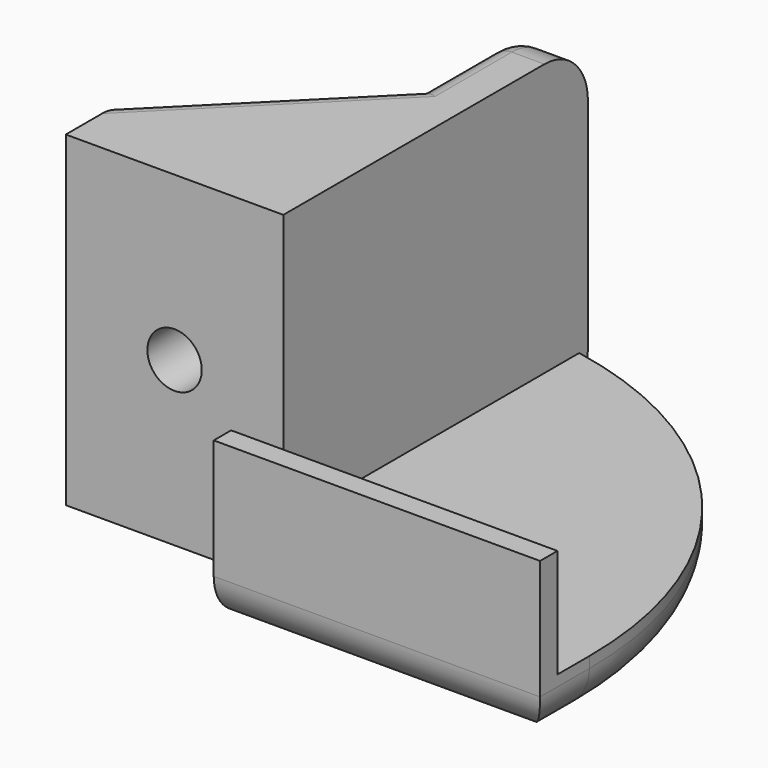
from build123d import *

# Parameters (mm, degrees)
F0_W          = 30
F0_H          = 42
F1_DEPTH      = 5
F2_T1_DEPTH   = 186.6590212458
F3_W          = 30
F3_H          = 2
F4_DEPTH      = 10
F5_W          = 35
F5_H          = 30
F6_DEPTH      = 5
F7_W          = 7
F7_H          = 30
F8_DEPTH      = 15
F9_R          = 2.5
F10_DEPTH     = 10
F11_R         = 4
F12_W         = 15
F12_H         = 14
F13_DEPTH     = 5
F14_W         = 15
F14_H         = 15
F15_DEPTH     = 5
F16_T4_DEPTH  = 35.8601958556
F16_T9_DEPTH  = 35.8601958556
F17_R         = 5
F18_T1_DEPTH  = 20
F18_T6_DEPTH  = 9.5699020722
F18_T11_DEPTH = 31.2132034356
F18_T16_DEPTH = 31.2132034356
F18_T21_DEPTH = 14
F18_T24_ANGLE = 90
F18_T26_ANGLE = 90
F18_T30_DEPTH = 13
F18_T36_DEPTH = 14
F18_T40_DEPTH = 31.2132034356
F18_T47_DEPTH = 13
F18_T51_DEPTH = 31.2132034356


# Not quite as in the source:
# - a fillet or chamfer that OpenCascade refuses, or shapes differently, is made with other operations: its cross-section is extruded or revolved along the edge and cut away or added


with BuildPart() as f1:
    # F0 (on Top) → F1 (new body)
    with BuildSketch(Plane.XY):
        with Locations((15, 21)):
            Rectangle(F0_W, F0_H)
    extrude(amount=F1_DEPTH)

    # F2: fillet of radius 37 on 1 edges, made by hand

    # F2_s2 → F2_t1 (cut)
    with BuildSketch(Plane.XY.offset(-90.8295106229)):
        with BuildLine():
            ThreePointArc((30, 5.6681957508), (21.5306852354, 29.2266337296), (0, 42))
            Line((0, 42), (30, 42))
            Line((30, 42), (30, 5.6681957508))
        make_face()
    extrude(amount=F2_T1_DEPTH, mode=Mode.SUBTRACT)

    # F3 (on face) → F4 (join)
    with BuildSketch(Plane.XY.offset(5)):
        with Locations((15, 1)):
            Rectangle(F3_W, F3_H)
    extrude(amount=F4_DEPTH)

    # F5 (on face) → F6 (join)
    with BuildSketch(Plane(origin=(0, 0, 0), x_dir=(0, -1, 0), z_dir=(-1, 0, 0))):
        with Locations((-25.5, 15)):
            Rectangle(F5_W, F5_H)
    extrude(amount=F6_DEPTH)

    # F7 (on face) → F8 (join)
    with BuildSketch(Plane(origin=(-5, 0, 0), x_dir=(0, -1, 0), z_dir=(-1, 0, 0))):
        with Locations((-11.5, 15)):
            Rectangle(F7_W, F7_H)
    extrude(amount=F8_DEPTH)

    # F9 (on face) → F10 (cut)
    with BuildSketch(Plane(origin=(0, 15, 0), x_dir=(-1, 0, 0), z_dir=(0, 1, 0))):
        with Locations((10, 15)):
            Circle(F9_R)
    extrude(amount=-F10_DEPTH, mode=Mode.SUBTRACT)

    # F11
    f11_edges = [f1.edges().sort_by_distance(p)[0] for p in [
        (21.530685, 29.226634, 0),
        (15, 0, 0),
    ]]
    fillet(f11_edges, radius=F11_R)

    # F12 (on face) → F13 (join)
    with BuildSketch(Plane(origin=(0, 0, 0), x_dir=(1, 0, 0), z_dir=(0, 0, -1))):
        with Locations((-12.5, -22)):
            Rectangle(F12_W, F12_H)
    extrude(amount=-F13_DEPTH)

    # F14 (on face) → F15 (join)
    with BuildSketch(Plane.XY.offset(30)):
        with Locations((-12.5, 22.5)):
            Rectangle(F14_W, F14_H)
    extrude(amount=-F15_DEPTH)

    # F16: chamfer of 15 on 2 edges, made by hand


with BuildPart() as f16_tool2:
    # F16_s3 → F16_t4 (new body)
    with BuildSketch(Plane.XY.offset(45.4300979278)):
        with BuildLine():
            Line((-20.4242640687, 14.5757359313), (-4.5757359313, 30.4242640687))
            Line((-4.5757359313, 30.4242640687), (-4.5757359313, 30.7242640687))
            ThreePointArc((-4.5757359313, 30.7242640687), (-12.2878679656, 30.3), (-20, 30.3))
            Line((-20, 30.3), (-20.3, 30))
            ThreePointArc((-20.3, 30), (-20.3, 22.2878679656), (-20.7242640687, 14.5757359313))
            Line((-20.7242640687, 14.5757359313), (-20.4242640687, 14.5757359313))
        make_face()
    extrude(amount=-F16_T4_DEPTH)

    split(bisect_by=Plane.YZ.offset(-5), keep=Keep.BOTTOM)


with BuildPart() as f1_1:
    add(f1.part)

    # F16_t1: cut F16_tool2
    add(f16_tool2.part, mode=Mode.SUBTRACT)


with BuildPart() as f16_tool7:
    # F16_s8 → F16_t9 (new body)
    with BuildSketch(Plane.XY.offset(-15.4300979278)):
        with BuildLine():
            Line((-4.5757359313, 29.4242640687), (-20.4242640687, 13.5757359313))
            Line((-20.4242640687, 13.5757359313), (-20.7242640687, 13.5757359313))
            ThreePointArc((-20.7242640687, 13.5757359313), (-20.3, 21.2878679656), (-20.3, 29))
            Line((-20.3, 29), (-20, 29.3))
            ThreePointArc((-20, 29.3), (-12.2878679656, 29.3), (-4.5757359313, 29.7242640687))
            Line((-4.5757359313, 29.7242640687), (-4.5757359313, 29.4242640687))
        make_face()
    extrude(amount=F16_T9_DEPTH)

    split(bisect_by=Plane.YZ.offset(-5), keep=Keep.BOTTOM)


with BuildPart() as f1_2:
    add(f1_1.part)

    # F16_t6: cut F16_tool7
    add(f16_tool7.part, mode=Mode.SUBTRACT)

    # F17
    f17_edges = [f1_2.edges().sort_by_distance(p)[0] for p in [
        (-2.5, 43, 0),
        (-2.5, 43, 30),
    ]]
    fillet(f17_edges, radius=F17_R)

    # F18: fillet of radius 2 on 9 edges, made by hand

    # F18_s2 → F18_t1 (cut)
    with BuildSketch(Plane.XY.offset(5)):
        with BuildLine():
            ThreePointArc((-3, 43), (-4.4142135624, 42.4142135624), (-5, 41))
            Line((-5, 41), (-5, 43))
            Line((-5, 43), (-3, 43))
        make_face()
    extrude(amount=F18_T1_DEPTH, mode=Mode.SUBTRACT)


with BuildPart() as f18_tool4:
    # F18_s5 → F18_t6 (new body)
    with BuildSketch(Plane.XY.offset(25)):
        with BuildLine():
            ThreePointArc((-20, 13), (-19.4142135624, 14.4142135624), (-18, 15))
            Line((-18, 15), (-20, 15))
            Line((-20, 15), (-20, 13))
        make_face()
    extrude(amount=-F18_T6_DEPTH)

    split(bisect_by=Plane(origin=(-17, 17, 0), x_dir=(0, 0, 1), z_dir=(-0.7071067812, 0.7071067812, 0)), keep=Keep.TOP)


with BuildPart() as f1_3:
    add(f1_2.part)

    # F18_t3: cut F18_tool4
    add(f18_tool4.part, mode=Mode.SUBTRACT)


with BuildPart() as f18_tool9:
    # F18_s10 → F18_t11 (new body)
    with BuildSketch(Plane(origin=(-6.5355339059, -6.5355339059, 0), x_dir=(0, 0, 1), z_dir=(0.7071067812, 0.7071067812, 0))):
        with BuildLine():
            ThreePointArc((0, -22.0416305603), (0.5857864376, -23.4558441227), (2, -24.0416305603))
            Line((2, -24.0416305603), (0, -24.0416305603))
            Line((0, -24.0416305603), (0, -22.0416305603))
        make_face()
    extrude(amount=F18_T11_DEPTH)

    split(bisect_by=Plane.YZ.offset(-5), keep=Keep.BOTTOM)


with BuildPart() as f1_4:
    add(f1_3.part)

    # F18_t8: cut F18_tool9
    add(f18_tool9.part, mode=Mode.SUBTRACT)


with BuildPart() as f18_tool14:
    # F18_s15 → F18_t16 (new body)
    with BuildSketch(Plane(origin=(16.0355339059, 16.0355339059, 0), x_dir=(0, 0, 1), z_dir=(-0.7071067812, -0.7071067812, 0))):
        with BuildLine():
            ThreePointArc((30, 22.7487373415), (29.4142135624, 24.1629509039), (28, 24.7487373415))
            Line((28, 24.7487373415), (30, 24.7487373415))
            Line((30, 24.7487373415), (30, 22.7487373415))
        make_face()
    extrude(amount=F18_T16_DEPTH)

    split(bisect_by=Plane.YZ.offset(-5), keep=Keep.BOTTOM)


with BuildPart() as f1_5:
    add(f1_4.part)

    # F18_t13: cut F18_tool14
    add(f18_tool14.part, mode=Mode.SUBTRACT)


with BuildPart() as f18_tool19:
    # F18_s20 → F18_t21 (new body)
    with BuildSketch(Plane.XZ.offset(-24)):
        with BuildLine():
            ThreePointArc((-3, 0), (-4.4142135624, 0.5857864376), (-5, 2))
            Line((-5, 2), (-5, 0))
            Line((-5, 0), (-3, 0))
        make_face()
    extrude(amount=-F18_T21_DEPTH)

    split(bisect_by=Plane(origin=(-17, 17, 0), x_dir=(0, 0, 1), z_dir=(-0.7071067812, 0.7071067812, 0)), keep=Keep.TOP)


with BuildPart() as f1_6:
    add(f1_5.part)

    # F18_t18: cut F18_tool19
    add(f18_tool19.part, mode=Mode.SUBTRACT)

    # F18_s23 → F18_t24 (revolve, cut)
    with BuildSketch(Plane.XY.offset(5)):
        with BuildLine():
            ThreePointArc((-3, 43), (-4.4142135624, 42.4142135624), (-5, 41))
            Line((-5, 41), (-5, 43))
            Line((-5, 43), (-3, 43))
        make_face()
    revolve(axis=Axis((-5, 38, 5), (-1, 0, 0)), revolution_arc=F18_T24_ANGLE, mode=Mode.SUBTRACT)

    # F18_s25 → F18_t26 (revolve, cut)
    with BuildSketch(Plane.XY.offset(25)):
        with BuildLine():
            ThreePointArc((-3, 43), (-4.4142135624, 42.4142135624), (-5, 41))
            Line((-5, 41), (-5, 43))
            Line((-5, 43), (-3, 43))
        make_face()
    revolve(axis=Axis((-5, 38, 25), (1, 0, 0)), revolution_arc=F18_T26_ANGLE, mode=Mode.SUBTRACT)


with BuildPart() as f18_tool28:
    # F18_s29 → F18_t30 (new body)
    with BuildSketch(Plane.XZ.offset(-25)):
        with BuildLine():
            ThreePointArc((-3, 30), (-4.4142135624, 29.4142135624), (-5, 28))
            Line((-5, 28), (-5, 30))
            Line((-5, 30), (-3, 30))
        make_face()
    extrude(amount=-F18_T30_DEPTH)

    split(bisect_by=Plane(origin=(-17.5, 17.5, 0), x_dir=(0, 0, 1), z_dir=(-0.7071067812, 0.7071067812, 0)), keep=Keep.TOP)


with BuildPart() as f1_7:
    add(f1_6.part)

    # F18_t27: cut F18_tool28
    add(f18_tool28.part, mode=Mode.SUBTRACT)


with BuildPart() as f18_tool34:
    # F18_s35 → F18_t36 (new body)
    with BuildSketch(Plane.XZ.offset(-24)):
        with BuildLine():
            ThreePointArc((-3, 0), (-4.4142135624, 0.5857864376), (-5, 2))
            Line((-5, 2), (-5, 0))
            Line((-5, 0), (-3, 0))
        make_face()
    extrude(amount=-F18_T36_DEPTH)

    split(bisect_by=Plane(origin=(-17, 17, 0), x_dir=(0, 0, 1), z_dir=(0.7071067812, -0.7071067812, 0)), keep=Keep.TOP)


with BuildPart() as f18_tool38:
    # F18_s39 → F18_t40 (new body)
    with BuildSketch(Plane(origin=(-6.5355339059, -6.5355339059, 0), x_dir=(0, 0, 1), z_dir=(0.7071067812, 0.7071067812, 0))):
        with BuildLine():
            ThreePointArc((0, -22.0416305603), (0.5857864376, -23.4558441227), (2, -24.0416305603))
            Line((2, -24.0416305603), (0, -24.0416305603))
            Line((0, -24.0416305603), (0, -22.0416305603))
        make_face()
    extrude(amount=F18_T40_DEPTH)

    split(bisect_by=Plane.YZ.offset(-5), keep=Keep.TOP)


with BuildPart() as f18_tool34_1:
    add(f18_tool34.part)

    # F18_t42: intersect F18_tool38
    add(f18_tool38.part, mode=Mode.INTERSECT)


with BuildPart() as f1_8:
    add(f1_7.part)

    # F18_t32: cut F18_tool34
    add(f18_tool34_1.part, mode=Mode.SUBTRACT)


with BuildPart() as f18_tool45:
    # F18_s46 → F18_t47 (new body)
    with BuildSketch(Plane.XZ.offset(-25)):
        with BuildLine():
            ThreePointArc((-3, 30), (-4.4142135624, 29.4142135624), (-5, 28))
            Line((-5, 28), (-5, 30))
            Line((-5, 30), (-3, 30))
        make_face()
    extrude(amount=-F18_T47_DEPTH)

    split(bisect_by=Plane(origin=(-17.5, 17.5, 0), x_dir=(0, 0, 1), z_dir=(0.7071067812, -0.7071067812, 0)), keep=Keep.TOP)


with BuildPart() as f18_tool49:
    # F18_s50 → F18_t51 (new body)
    with BuildSketch(Plane(origin=(16.0355339059, 16.0355339059, 0), x_dir=(0, 0, 1), z_dir=(-0.7071067812, -0.7071067812, 0))):
        with BuildLine():
            ThreePointArc((30, 22.7487373415), (29.4142135624, 24.1629509039), (28, 24.7487373415))
            Line((28, 24.7487373415), (30, 24.7487373415))
            Line((30, 24.7487373415), (30, 22.7487373415))
        make_face()
    extrude(amount=F18_T51_DEPTH)

    split(bisect_by=Plane.YZ.offset(-5), keep=Keep.TOP)


with BuildPart() as f18_tool45_1:
    add(f18_tool45.part)

    # F18_t53: intersect F18_tool49
    add(f18_tool49.part, mode=Mode.INTERSECT)


with BuildPart() as f1_9:
    add(f1_8.part)

    # F18_t43: cut F18_tool45
    add(f18_tool45_1.part, mode=Mode.SUBTRACT)


solid = f1_9.part
